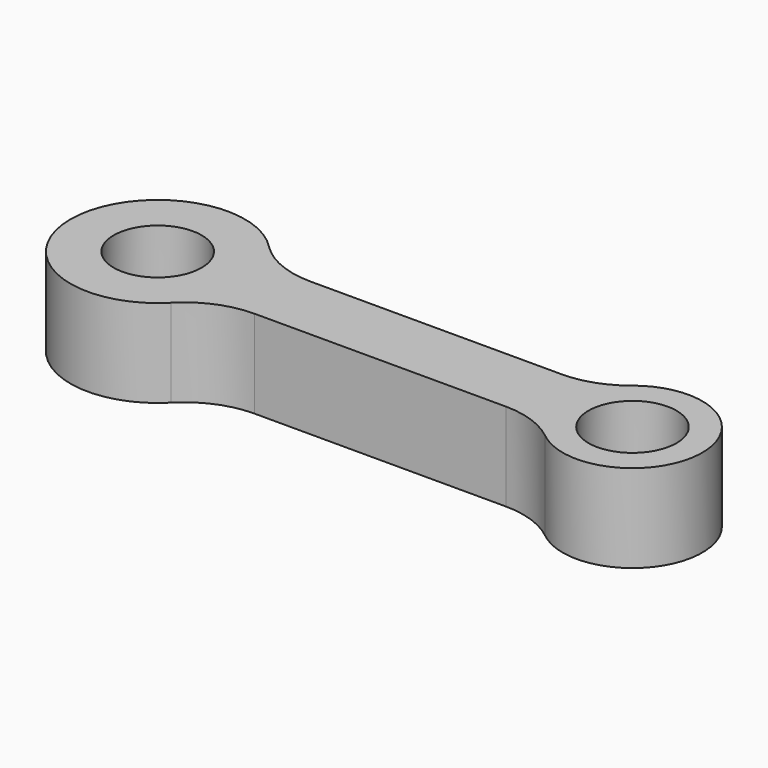
from build123d import *

# Parameters (mm, degrees)
F0_R     = 1.6002
F1_DEPTH = 3.2004


# Not quite as in the source:
# - ends of sketch curves that miss each other by under 0.0002 mm in the source are joined


with BuildPart() as f1:
    # F0 (on Top) → F1 (new body)
    with BuildSketch(Plane.XY):
        with BuildLine():
            ThreePointArc((-4.1050543049, 1.270002348), (-5.3326449309, 1.5185429247), (-6.3685964739, 2.2225))
            ThreePointArc((-6.3685964739, 2.2225), (-11.811, 0), (-6.3685964739, -2.2225))
            ThreePointArc((-6.3685964739, -2.2225), (-5.3326449309, -1.5185429247), (-4.1050543049, -1.270002348))
            Line((-4.1050543049, -1.270002348), (-4.1011929479, -1.27))
            Line((-4.1011929479, -1.27), (5.0438975516, -1.27))
            ThreePointArc((5.0438975516, -1.27), (6.1022308849, -1.451581293), (7.0395100229, -1.9755555556))
            ThreePointArc((7.0395100229, -1.9755555556), (11.176, 0), (7.0395100229, 1.9755555556))
            ThreePointArc((7.0395100229, 1.9755555556), (6.1022308849, 1.451581293), (5.0438975516, 1.27))
            Line((5.0438975516, 1.27), (-4.1011929479, 1.27))
            Line((-4.1011929479, 1.27), (-4.1050543049, 1.270002348))
        make_face()
        with Locations((-8.636, 0)):
            Circle(F0_R, mode=Mode.SUBTRACT)
        with Locations((8.636, 0)):
            Circle(F0_R, mode=Mode.SUBTRACT)
    extrude(amount=F1_DEPTH)


solid = f1.part
